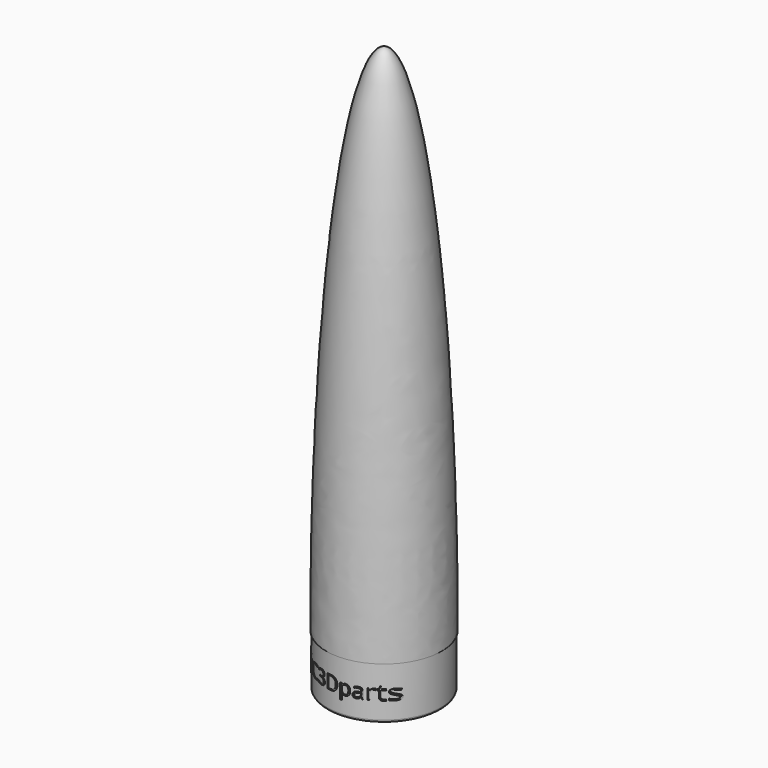
from build123d import *

# Parameters (mm, degrees)
F3_TEXT_SIZE = 11.1111111111
F5_DEPTH     = 38
F4_W         = 32
F4_H         = 38.2836783878
F9_R         = 1.5


# Not quite as in the source:
# - Text() gives the source's letters only with a copy of the font that has no kerning and outlines rounded to 1/6400 em; it was checked with that copy


with BuildPart() as f1:
    # F0 (on Front) → F1 (revolve)
    with BuildSketch(Plane.XZ):
        with BuildLine():
            Line((0, -30), (0, 294))
            add(Edge.make_bspline(
                [(0, 294), (-33, 294), (-33, 0)],
                knots=[0, 0, 0, 1.5707963268, 1.5707963268, 1.5707963268], degree=2, weights=[1, 0.7071067812, 1]))
            Line((-33, 0), (-32.55, 0))
            Line((-32.55, 0), (-32.55, -30))
            Line((-32.55, -30), (0, -30))
        make_face()
    revolve(axis=Axis((0, 0, 0), (0, 0, -1)))


with BuildPart() as f5:
    # F3 (on offset) → F5 (new body)
    with BuildSketch(Plane.XZ.offset(40)):
        with Locations((-29.5510814618, -18.7571294363)):
            Text('DC3Dparts', F3_TEXT_SIZE, font='Open Sans', text_align=(TextAlign.LEFT, TextAlign.BOTTOM))
    extrude(amount=-F5_DEPTH)


with BuildPart() as f6:
    # F4 (on Front) → F6 (revolve)
    with BuildSketch(Plane.XZ):
        with Locations((-16, -28.2593530889)):
            Rectangle(F4_W, F4_H)
    revolve(axis=Axis((0, 0, -28.2593530889), (0, 0, -1)))


with BuildPart() as f5_1:
    add(f5.part)

    # F7: cut F6
    add(f6.part, mode=Mode.SUBTRACT)


with BuildPart() as f1_1:
    add(f1.part)

    # F8: cut F5
    add(f5_1.part, mode=Mode.SUBTRACT)

    # F9
    f9_edges = [f1_1.edges().sort_by_distance(p)[0] for p in [
        (32.55, 0, -30),
    ]]
    fillet(f9_edges, radius=F9_R)


solid = f1_1.part
